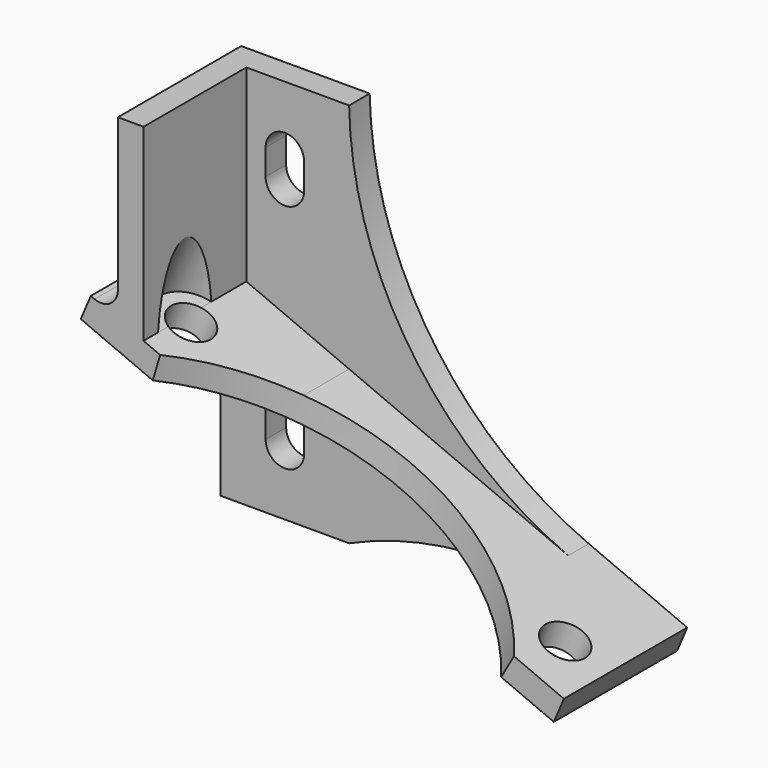
from build123d import *

# Parameters (mm, degrees)
F0_W          = 10
F0_H          = 30
F1_DEPTH      = 2
F3_DEPTH      = 10
F3_DEPTH_BACK = 2
F4_R          = 1.5
F4_R_2        = 19
F5_DEPTH      = 28.2830263058
F5_TAPER      = -5
F6_R          = 2.65
F7_DEPTH      = 55
F8_T1_DEPTH   = 2


# Not quite as in the source:
# - a fillet or chamfer that OpenCascade refuses, or shapes differently, is made with other operations: its cross-section is extruded or revolved along the edge and cut away or added
# - an extrude ends at something that could not be found from the text; its depth is read off the source's solid
# - a feature names something its author has since deleted; it is built from what else it names


with BuildPart() as f1:
    # F0 (on Front) → F1 (new body)
    with BuildSketch(Plane.XZ):
        with Locations((0, 4.7131987304)):
            Rectangle(F0_W, F0_H)
        with BuildLine():
            ThreePointArc((-1.5, -3.2868012696), (0, -1.7868012696), (1.5, -3.2868012696))
            Line((1.5, -3.2868012696), (1.5, -5.2868012696))
            ThreePointArc((1.5, -5.2868012696), (0, -6.7868012696), (-1.5, -5.2868012696))
            Line((-1.5, -5.2868012696), (-1.5, -3.2868012696))
        make_face(mode=Mode.SUBTRACT)
        with BuildLine():
            ThreePointArc((-1.5, 14.7131987304), (0, 16.2131987304), (1.5, 14.7131987304))
            Line((1.5, 14.7131987304), (1.5, 12.7131987304))
            ThreePointArc((1.5, 12.7131987304), (0, 11.2131987304), (-1.5, 12.7131987304))
            Line((-1.5, 12.7131987304), (-1.5, 14.7131987304))
        make_face(mode=Mode.SUBTRACT)
    extrude(amount=F1_DEPTH)

    # F2 (on face) → F3 (join, two sides)
    with BuildSketch(Plane.XZ.offset(2)) as f3_sk:
        with BuildLine():
            Line((-7.8870679483, 4.9496821465), (-5, 3.7241945098))
            Line((-5, 3.7241945098), (-5, 7.8610010163))
            ThreePointArc((-5, 7.8610010163), (-5.5824819191, 6.7769494476), (-6.807950467, 6.6643447068))
            Line((-6.807950467, 6.6643447068), (-7.1056056914, 6.7906918534))
            Line((-7.1056056914, 6.7906918534), (-7.8870679483, 4.9496821465))
        make_face()
        Polygon((5, -0.5205536523), (28.9331261898, -10.679562993), (29.7145884467, -8.8385532861), (5, 1.6521671025), align=None)
        Polygon((-5, 3.7241945098), (5, -0.5205536523), (5, 1.6521671025), (-3, 5.0479656322), (-3, 19.7131987304), (-5, 19.7131987304), (-5, 7.8610010163), align=None)
    extrude(amount=F3_DEPTH)
    extrude(f3_sk.sketch, amount=-F3_DEPTH_BACK)

    # F4 (on face) → F5 (cut, through all)
    with BuildSketch(Plane(origin=(0.5761265937, 0, 1.3572691988), x_dir=(0.9205048535, 0, -0.3907311285), z_dir=(-0.3907311285, 0, -0.9205048535))):
        with Locations((-4.1940792167, 8)):
            Circle(F4_R)
        with Locations((27.4445048224, 8)):
            Circle(F4_R)
        with Locations((11.6252128028, 24)):
            Circle(F4_R_2)
    extrude(amount=-F5_DEPTH, taper=F5_TAPER, mode=Mode.SUBTRACT)

    # F6 (on face) → F7 (cut, through all)
    with BuildSketch(Plane(origin=(1.3575888507, 0, 3.1982789057), x_dir=(0.9205048535, 0, -0.3907311285), z_dir=(0.3907311285, 0, 0.9205048535))):
        with Locations((27.4445048224, -8)):
            Circle(F6_R)
        with Locations((-4.1940792167, -8)):
            Circle(F6_R)
    extrude(amount=F7_DEPTH, mode=Mode.SUBTRACT)

    # F8: fillet of radius 28 on 2 edges, made by hand

    # F8_s2 → F8_t1 (join)
    with BuildSketch(Plane.XZ):
        with BuildLine():
            ThreePointArc((22.0555251238, -5.5874737898), (9.7786939327, 4.5355646625), (5, 19.7131987304))
            Line((5, 19.7131987304), (5, 1.6521671025))
            Line((5, 1.6521671025), (22.0555251238, -5.5874737898))
        make_face()
        with BuildLine():
            ThreePointArc((27.43600386, -10.0440722673), (16.1926256307, -7.8198466481), (5, -10.2868012696))
            Line((5, -10.2868012696), (5, -0.5205536523))
            Line((5, -0.5205536523), (27.43600386, -10.0440722673))
        make_face()
    extrude(amount=F8_T1_DEPTH)


solid = f1.part
